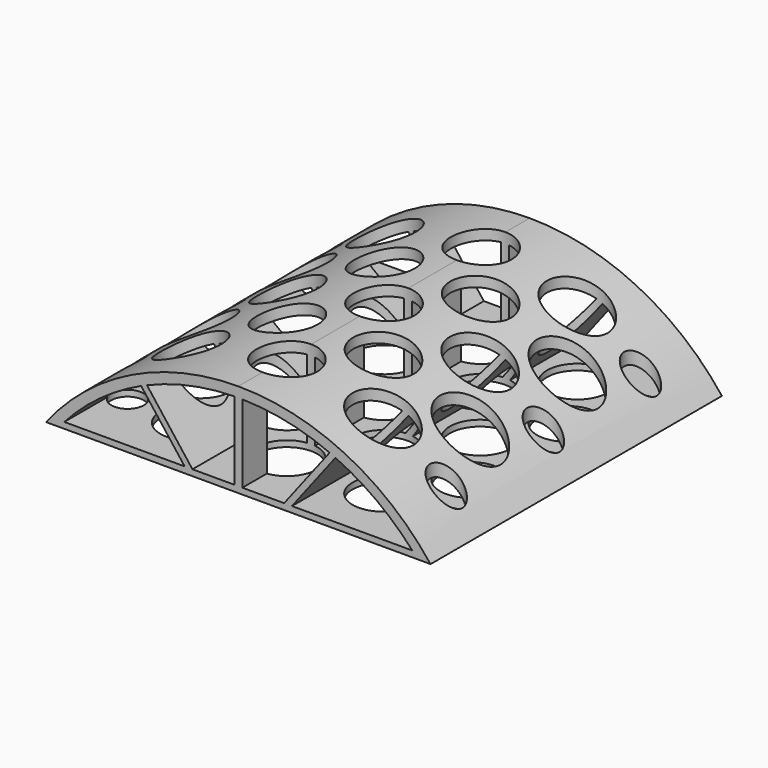
from build123d import *
from build123d import SkipClean  # not in build123d's __all__

# Parameters (mm, degrees)
F1_DEPTH = 90
F2_R     = 4
F2_R_2   = 7.5
F3_DEPTH = 30


with BuildPart() as f1:
    # F0 (on Front) → F1 (new body)
    with BuildSketch(Plane.XZ):
        with BuildLine():
            Line((-1, 0), (0, 0))
            Line((0, 0), (1, 0))
            Line((1, 0), (4.75, 0))
            Line((4.75, 0), (47.5, 0))
            ThreePointArc((47.5, 0), (26.4391835898, 17.115114603), (0, 23.2351396719))
            ThreePointArc((0, 23.2351396719), (-26.4391835898, 17.115114603), (-47.5, 0))
            Line((-47.5, 0), (-1, 0))
        make_face()
        with BuildLine():
            Line((-24.0064691199, 15.5010001914), (-13.2575714961, 1.5))
            Line((-13.2575714961, 1.5), (-42.9952852877, 1.5))
            ThreePointArc((-42.9952852877, 1.5), (-34.2244908656, 9.4818990396), (-24.0064691199, 15.5010001914))
        make_face(mode=Mode.SUBTRACT)
        with BuildLine():
            Line((-1, 20.7264690173), (-1, 1.5))
            Line((-1, 1.5), (-11.3296266645, 1.5))
            Line((-11.3296266645, 1.5), (-22.5665086085, 16.1366252387))
            ThreePointArc((-22.5665086085, 16.1366252387), (-12.0046552835, 19.4718540221), (-1, 20.7264690173))
        make_face(mode=Mode.SUBTRACT)
        with BuildLine():
            Line((11.3296266645, 1.5), (1, 1.5))
            Line((1, 1.5), (1, 20.7264690173))
            ThreePointArc((1, 20.7264690173), (12.0046552835, 19.4718540221), (22.5665086085, 16.1366252387))
            Line((22.5665086085, 16.1366252387), (11.3296266645, 1.5))
        make_face(mode=Mode.SUBTRACT)
        with BuildLine():
            ThreePointArc((24.0064691199, 15.5010001914), (34.2244908656, 9.4818990396), (42.9952852877, 1.5))
            Line((42.9952852877, 1.5), (13.2575714961, 1.5))
            Line((13.2575714961, 1.5), (24.0064691199, 15.5010001914))
        make_face(mode=Mode.SUBTRACT)
    extrude(amount=F1_DEPTH)

    # F2 (on face) → F3 (cut)
    with BuildSketch(Plane(origin=(0, 0, 0), x_dir=(1, 0, 0), z_dir=(0, 0, -1))):
        with Locations((-39.375, 75)):
            Circle(F2_R)
        with Locations((-23.75, 75)):
            Circle(F2_R_2)
        with Locations((0, 75)):
            Circle(F2_R_2)
        with Locations((23.75, 75)):
            Circle(F2_R_2)
        with Locations((39.375, 75)):
            Circle(F2_R)
        with Locations((-33.3125, 60)):
            Circle(F2_R_2)
        with Locations((-11.875, 60)):
            Circle(F2_R_2)
        with Locations((11.875, 60)):
            Circle(F2_R_2)
        with Locations((33.3125, 60)):
            Circle(F2_R_2)
        with Locations((39.375, 45)):
            Circle(F2_R)
        with Locations((23.75, 45)):
            Circle(F2_R_2)
        with Locations((0, 45)):
            Circle(F2_R_2)
        with Locations((-23.75, 45)):
            Circle(F2_R_2)
        with Locations((-39.375, 45)):
            Circle(F2_R)
        with Locations((-33.3125, 30)):
            Circle(F2_R_2)
        with Locations((-11.875, 30)):
            Circle(F2_R_2)
        with Locations((11.875, 30)):
            Circle(F2_R_2)
        with Locations((33.3125, 30)):
            Circle(F2_R_2)
        with Locations((39.375, 15)):
            Circle(F2_R)
        with Locations((23.75, 15)):
            Circle(F2_R_2)
        with Locations((0, 15)):
            Circle(F2_R_2)
        with Locations((-23.75, 15)):
            Circle(F2_R_2)
        with Locations((-39.375, 15)):
            Circle(F2_R)
    with SkipClean():  # cleaning this boolean's faces spoils the solid; the shape is the same uncleaned
        extrude(amount=-F3_DEPTH, mode=Mode.SUBTRACT)


solid = f1.part
